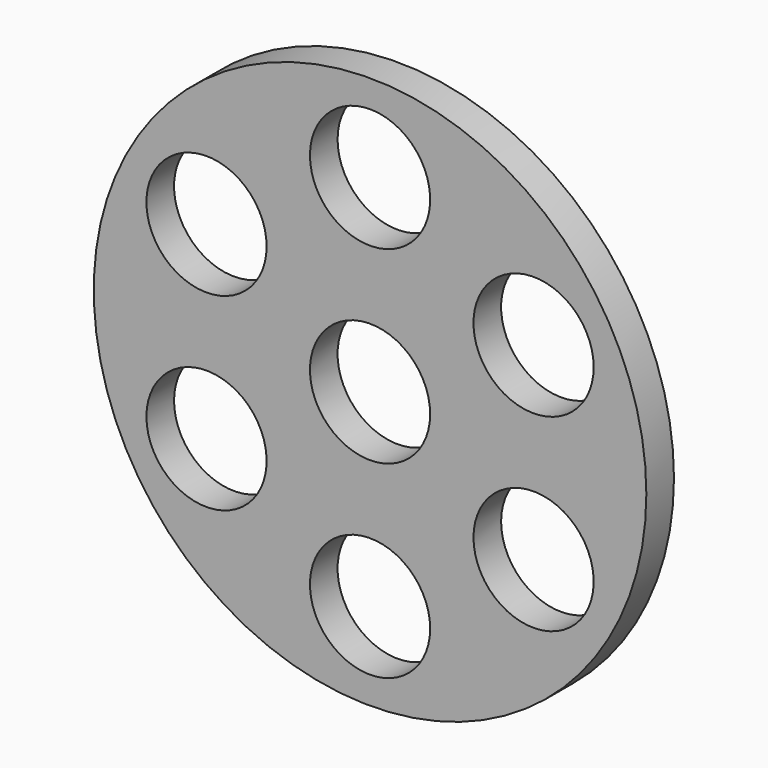
from build123d import *

# Parameters (mm, degrees)
F0_R            = 50.8
F2_DEPTH        = 6.35
F1_R            = 11.049
F3_DEPTH        = 10.414
F5_R            = 11.049
F6_DEPTH        = 6.35
F6_COPIES_COUNT = 6


# Not quite as in the source:
# - a pattern or mirror of a feature is missing from the dataset's text; its kind, count and spacing are read off the source's solid
# - a feature names something its author has since deleted; it is built from what else it names


with BuildPart() as f2:
    # F0 (on Front) → F2 (new body)
    with BuildSketch(Plane.XZ):
        Circle(F0_R)
    extrude(amount=F2_DEPTH)

    # F1 (on Front) → F3 (cut)
    with BuildSketch(Plane.XZ):
        Circle(F1_R)
    extrude(amount=F3_DEPTH, mode=Mode.SUBTRACT)

    # F5 (on Front) → F6 (cut)
    with BuildSketch(Plane.XZ):
        with Locations((0, -34.7183458507)):
            Circle(F5_R)
    f6 = extrude(amount=F6_DEPTH, mode=Mode.SUBTRACT)

    # F6_copies: F6 ×6 about axis
    f6_copies_axis = Axis((0, 0, 0), (0, 1, 0))
    for i in range(1, F6_COPIES_COUNT):
        add(f6.rotate(f6_copies_axis, i * 360 / F6_COPIES_COUNT), mode=Mode.SUBTRACT)


solid = f2.part
